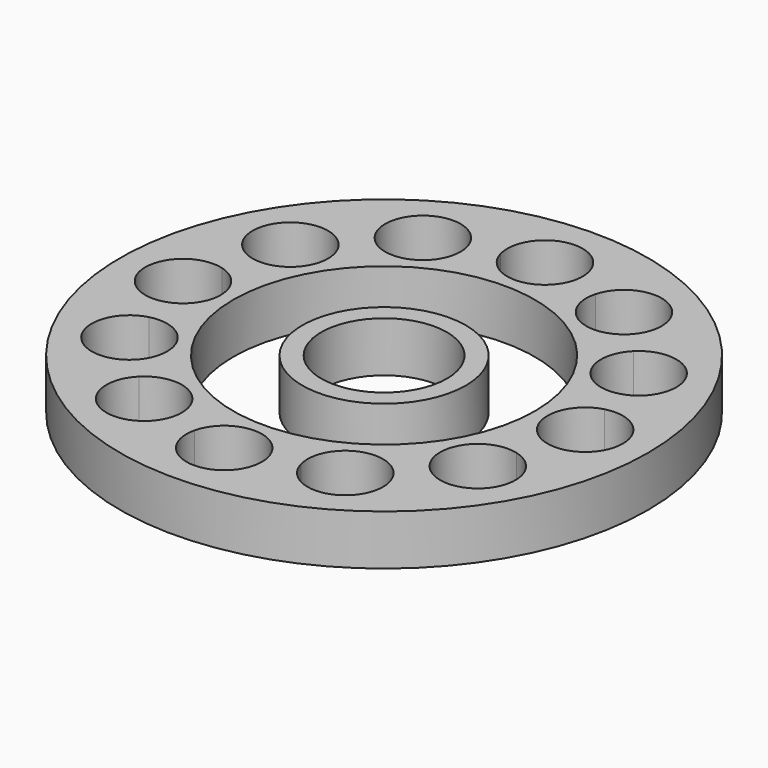
from build123d import *

# Parameters (mm, degrees)
F0_R     = 10.5
F0_R_2   = 6
F1_DEPTH = 2
F0_R_3   = 3.25
F0_R_4   = 2.5


# Not quite as in the source:
# - the program builds the solid bodies; features that only make, move or delete a surface that nothing else refers to are left out


with BuildPart() as f1:
    # F0 (on Top) → F1 (new body)
    with BuildSketch(Plane.XY):
        Circle(F0_R)
        with BuildLine():
            ThreePointArc((-5.0606601718, 5.8675430585), (-4.75, 8.227241336), (-2.5511112606, 7.3164317979))
            Line((-2.5511112606, 7.3164317979), (-1.4488887394, 7.6117714323))
            ThreePointArc((-1.4488887394, 7.6117714323), (-0.1957892883, 9.4871672921), (1.5, 8))
            ThreePointArc((1.5, 8), (1.4871672921, 7.8042107117), (1.4488887394, 7.6117714323))
            Line((1.4488887394, 7.6117714323), (2.5511112606, 7.3164317979))
            ThreePointArc((2.5511112606, 7.3164317979), (4.1957892883, 8.4153705223), (5.5, 6.9282032303))
            ThreePointArc((5.5, 6.9282032303), (5.3858192988, 6.3541780817), (5.0606601718, 5.8675430585))
            Line((5.0606601718, 5.8675430585), (5.8675430585, 5.0606601718))
            ThreePointArc((5.8675430585, 5.0606601718), (7.5022283788, 5.3858192988), (8.4282032303, 4))
            ThreePointArc((8.4282032303, 4), (8.1182332407, 3.0868578565), (7.3164317979, 2.5511112606))
            Line((7.3164317979, 2.5511112606), (7.6117714323, 1.4488887394))
            ThreePointArc((7.6117714323, 1.4488887394), (8.9131421435, 1.1900300104), (9.5, 0))
            ThreePointArc((9.5, 0), (8.9131421435, -1.1900300104), (7.6117714323, -1.4488887394))
            Line((7.6117714323, -1.4488887394), (7.3164317979, -2.5511112606))
            ThreePointArc((7.3164317979, -2.5511112606), (8.1182332407, -3.0868578565), (8.4282032303, -4))
            ThreePointArc((8.4282032303, -4), (7.5022283788, -5.3858192988), (5.8675430585, -5.0606601718))
            Line((5.8675430585, -5.0606601718), (5.0606601718, -5.8675430585))
            ThreePointArc((5.0606601718, -5.8675430585), (5.3858192988, -6.3541780817), (5.5, -6.9282032303))
            ThreePointArc((5.5, -6.9282032303), (4.1957892883, -8.4153705223), (2.5511112606, -7.3164317979))
            Line((2.5511112606, -7.3164317979), (1.4675350544, -7.6067751673))
            ThreePointArc((1.4675350544, -7.6067751673), (1.4996006084, -7.7833853166), (1.51034039, -7.9625612125))
            ThreePointArc((1.51034039, -7.9625612125), (-0.16617732, -9.4521388365), (-1.4481149408, -7.6119787711))
            Line((-1.4481149408, -7.6119787711), (-2.5504401106, -7.316611632))
            ThreePointArc((-2.5504401106, -7.316611632), (-4.7496981342, -8.2301088879), (-5.0593126587, -5.8688905716))
            Line((-5.0593126587, -5.8688905716), (-5.8675430585, -5.0606601718))
            ThreePointArc((-5.8675430585, -5.0606601718), (-8.227241336, -4.75), (-7.3164317979, -2.5511112606))
            Line((-7.3164317979, -2.5511112606), (-7.6117714323, -1.4488887394))
            ThreePointArc((-7.6117714323, -1.4488887394), (-9.5, 0), (-7.6117714323, 1.4488887394))
            Line((-7.6117714323, 1.4488887394), (-7.3164317979, 2.5511112606))
            ThreePointArc((-7.3164317979, 2.5511112606), (-8.227241336, 4.75), (-5.8675430585, 5.0606601718))
            Line((-5.8675430585, 5.0606601718), (-5.0606601718, 5.8675430585))
        make_face(mode=Mode.SUBTRACT)
        with BuildLine():
            ThreePointArc((-2.5511112606, 7.3164317979), (-2.5128327079, 7.1239925186), (-2.5, 6.9282032303))
            ThreePointArc((-2.5, 6.9282032303), (-3.4259748515, 5.5423839315), (-5.0606601718, 5.8675430585))
            Line((-5.0606601718, 5.8675430585), (-5.8675430585, 5.0606601718))
            ThreePointArc((-5.8675430585, 5.0606601718), (-5.5423839315, 4.5740251485), (-5.4282032303, 4))
            ThreePointArc((-5.4282032303, 4), (-6.0150610868, 2.8099699896), (-7.3164317979, 2.5511112606))
            Line((-7.3164317979, 2.5511112606), (-7.6117714323, 1.4488887394))
            ThreePointArc((-7.6117714323, 1.4488887394), (-6.8099699896, 0.9131421435), (-6.5, 0))
            ThreePointArc((-6.5, 0), (-6.8099699896, -0.9131421435), (-7.6117714323, -1.4488887394))
            Line((-7.6117714323, -1.4488887394), (-7.3164317979, -2.5511112606))
            ThreePointArc((-7.3164317979, -2.5511112606), (-6.0150610868, -2.8099699896), (-5.4282032303, -4))
            ThreePointArc((-5.4282032303, -4), (-5.5423839315, -4.5740251485), (-5.8675430585, -5.0606601718))
            Line((-5.8675430585, -5.0606601718), (-5.0593126587, -5.8688905716))
            ThreePointArc((-5.0593126587, -5.8688905716), (-3.4250952201, -5.5454419303), (-2.5, -6.9308965467))
            ThreePointArc((-2.5, -6.9308965467), (-2.5126634822, -7.1253961173), (-2.5504401106, -7.316611632))
            Line((-2.5504401106, -7.316611632), (-1.4481149408, -7.6119787711))
            ThreePointArc((-1.4481149408, -7.6119787711), (0.007663322, -6.4625636014), (1.4675350544, -7.6067751673))
            Line((1.4675350544, -7.6067751673), (2.5511112606, -7.3164317979))
            ThreePointArc((2.5511112606, -7.3164317979), (3.25, -5.6291651246), (5.0606601718, -5.8675430585))
            Line((5.0606601718, -5.8675430585), (5.8675430585, -5.0606601718))
            ThreePointArc((5.8675430585, -5.0606601718), (5.6291651246, -3.25), (7.3164317979, -2.5511112606))
            Line((7.3164317979, -2.5511112606), (7.6117714323, -1.4488887394))
            ThreePointArc((7.6117714323, -1.4488887394), (6.5, 0), (7.6117714323, 1.4488887394))
            Line((7.6117714323, 1.4488887394), (7.3164317979, 2.5511112606))
            ThreePointArc((7.3164317979, 2.5511112606), (5.6291651246, 3.25), (5.8675430585, 5.0606601718))
            Line((5.8675430585, 5.0606601718), (5.0606601718, 5.8675430585))
            ThreePointArc((5.0606601718, 5.8675430585), (3.25, 5.6291651246), (2.5511112606, 7.3164317979))
            Line((2.5511112606, 7.3164317979), (1.4488887394, 7.6117714323))
            ThreePointArc((1.4488887394, 7.6117714323), (0, 6.5), (-1.4488887394, 7.6117714323))
            Line((-1.4488887394, 7.6117714323), (-2.5511112606, 7.3164317979))
        make_face()
        Circle(F0_R_2, mode=Mode.SUBTRACT)
    extrude(amount=F1_DEPTH)


with BuildPart() as f1b:
    # F0 (on Top) → F1, piece 2 (new body)
    with BuildSketch(Plane.XY):
        Circle(F0_R_3)
        Circle(F0_R_4, mode=Mode.SUBTRACT)
    extrude(amount=F1_DEPTH)


solid = Compound([f1.part, f1b.part])
